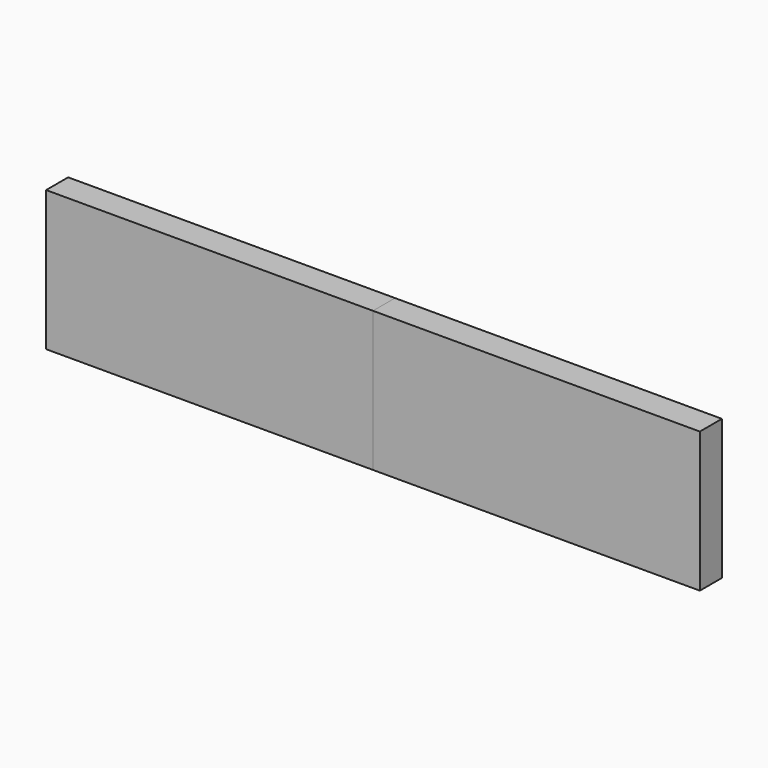
from build123d import *

# Parameters (mm, degrees)
F0_W     = 177.8
F0_H     = 76.2
F1_DEPTH = 15


with BuildPart() as f1:
    # F0 (on Front) → F1 (new body)
    with BuildSketch(Plane.XZ):
        with Locations((-5.625751482, 17.6829374395)):
            Rectangle(F0_W, F0_H)
    extrude(amount=F1_DEPTH)


with BuildPart() as f2_1:
    # F2: copy of F1
    add(f1.part.moved(Location((-177.8, 0, 0))))


solid = Compound([f1.part, f2_1.part])
